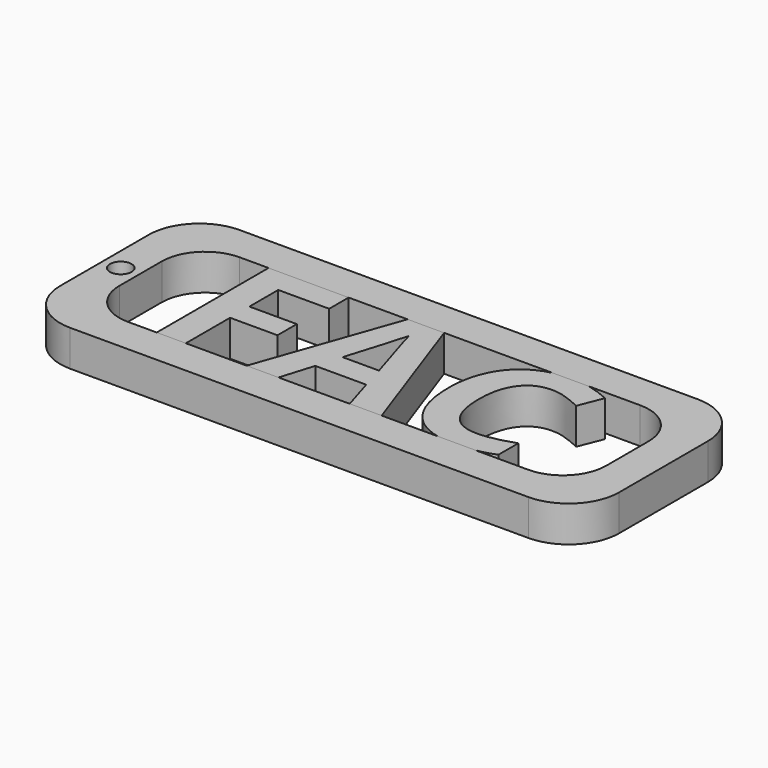
from build123d import *

# Parameters (mm, degrees)
F0_TEXT_SIZE = 27.1600746902
F1_DEPTH     = 5
F2_W         = 77.5598370396
F2_H         = 29.3897470718
F2_W_2       = 67.5598370396
F2_H_2       = 19.3897470718
F3_DEPTH     = 5
F4_R         = 6
F5_R         = 7
F6_R         = 1.5
F7_DEPTH     = 5.0010001


# Not quite as in the source:
# - Text() gives the source's letters only with a copy of the font that has no kerning and outlines rounded to 1/6400 em; it was checked with that copy


with BuildPart() as f1:
    # F0 (on Top) → F1 (new body)
    with BuildSketch(Plane.XY):
        with Locations((0, -19.5552537769)):
            Text('FAC', F0_TEXT_SIZE, font='Open Sans', font_style=FontStyle.BOLD, text_align=(TextAlign.LEFT, TextAlign.BOTTOM))
    extrude(amount=-F1_DEPTH)


with BuildPart() as f3:
    # F2 (on Top) → F3 (new body)
    with BuildSketch(Plane.XY):
        with Locations((26.2200814802, -9.860380241)):
            Rectangle(F2_W, F2_H)
        with Locations((26.2200814802, -9.860380241)):
            Rectangle(F2_W_2, F2_H_2, mode=Mode.SUBTRACT)
    extrude(amount=-F3_DEPTH)

    # F4
    f4_edges = [f3.edges().sort_by_distance(p)[0] for p in [
        (-7.559837, -0.165507, -2.5),
        (-7.559837, -19.555254, -2.5),
        (60, -0.165507, -2.5),
        (60, -19.555254, -2.5),
    ]]
    fillet(f4_edges, radius=F4_R)

    # F5
    f5_edges = [f3.edges().sort_by_distance(p)[0] for p in [
        (-12.559837, 4.834493, -2.5),
        (-12.559837, -24.555254, -2.5),
        (65, 4.834493, -2.5),
        (65, -24.555254, -2.5),
    ]]
    fillet(f5_edges, radius=F5_R)

    # F6 (on face) → F7 (cut, through all)
    with BuildSketch(Plane.XY):
        with Locations((-10.0598370396, -10.1655067051)):
            Circle(F6_R)
    extrude(amount=-F7_DEPTH, mode=Mode.SUBTRACT)


solid = Compound([f1.part, f3.part])
